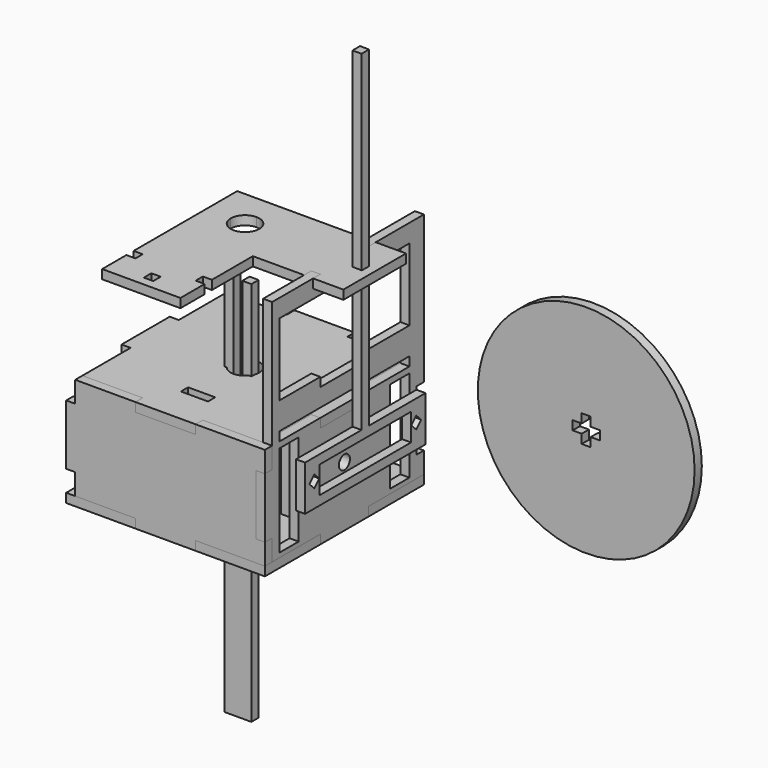
from build123d import *

# Parameters (mm, degrees)
F0_W      = 3
F0_H      = 10
F0_R      = 4.75
F1_DEPTH  = 3
F2_W      = 8
F2_H      = 30.5
F2_R      = 2.3
F2_W_2    = 20
F2_H_2    = 3
F2_W_3    = 3
F2_H_3    = 20
F3_DEPTH  = 3
F5_DEPTH  = 3
F6_R      = 4.75
F6_W      = 20
F6_H      = 3
F6_W_2    = 3
F6_H_2    = 20
F7_DEPTH  = 3
F8_W      = 3
F8_H      = 20
F8_W_2    = 20
F8_H_2    = 3
F8_H_3    = 7
F9_DEPTH  = 3
F10_W     = 17
F10_H     = 20
F10_H_2   = 3
F10_W_2   = 3
F10_W_3   = 3.125
F10_H_3   = 3.125
F10_H_4   = 17
F11_DEPTH = 3
F12_W     = 3.125
F12_H     = 110
F12_W_2   = 6
F12_H_2   = 9
F13_DEPTH = 3
F14_R     = 36
F15_DEPTH = 3
F17_DEPTH = 3
F18_W     = 3
F18_H     = 9
F18_W_2   = 9
F18_H_2   = 3
F19_DEPTH = 37
F20_R     = 2.3
F20_W     = 9
F20_H     = 3
F21_DEPTH = 3


with BuildPart() as f1:
    # F0 (on Top) → F1 (new body)
    with BuildSketch(Plane.XY):
        Polygon((33, 10), (33, 33), (10, 33), (10, 30), (-10, 30), (-10, 33), (-33, 33), (-33, 10), (-30, 10), (-30, -10), (-33, -10), (-33, -33), (-10, -33), (-10, -30), (10, -30), (10, -33), (33, -33), (33, -10), (30, -10), (30, 10), align=None)
        with Locations((-10, 0)):
            Rectangle(F0_W, F0_H, mode=Mode.SUBTRACT)
        Circle(F0_R, mode=Mode.SUBTRACT)
        with Locations((10, 0)):
            Rectangle(F0_W, F0_H, mode=Mode.SUBTRACT)
    extrude(amount=F1_DEPTH)


with BuildPart() as f3:
    # F2 (on face) → F3 (new body)
    with BuildSketch(Plane.YZ.offset(30)):
        Polygon((-30, 10), (-30, 3), (-10, 3), (10, 3), (24, 3), (27, 3), (33, 3), (33, 10), (30, 10), (30, 30), (33, 30), (33, 37), (27, 37), (24, 37), (10, 37), (10, 34), (-10, 34), (-10, 37), (-24, 37), (-27, 37), (-30, 37), (-30, 30), align=None)
        with Locations((-23, 19.75)):
            Rectangle(F2_W, F2_H, mode=Mode.SUBTRACT)
        with Locations((0, 20)):
            Circle(F2_R, mode=Mode.SUBTRACT)
        with Locations((23, 19.75)):
            Rectangle(F2_W, F2_H, mode=Mode.SUBTRACT)
        with Locations((0, 1.5)):
            Rectangle(F2_W_2, F2_H_2)
        with Locations((-31.5, 20)):
            Rectangle(F2_W_3, F2_H_3)
        Polygon((-30, 79), (-30, 49), (-27, 49), (-27, 73), (27, 73), (27, 49), (33, 49), (33, 79), (10, 79), (10, 76), (-10, 76), (-10, 79), align=None)
        Polygon((-30, 49), (-30, 37), (-27, 37), (-27, 40), (27, 40), (27, 37), (33, 37), (33, 49), (27, 49), (10, 49), (10, 46), (-10, 46), (-10, 49), (-27, 49), align=None)
    extrude(amount=F3_DEPTH)


with BuildPart() as f5:
    # F4 (on Front) → F5 (new body)
    with BuildSketch(Plane.XZ):
        Polygon((4.5, -64), (4.5, 64), (1.5, 64), (1.5, 0), (-1.5, 0), (-1.5, 64), (-4.5, 64), (-4.5, -64), align=None)
    extrude(amount=F5_DEPTH)


with BuildPart() as f7:
    # F6 (on face) → F7 (new body)
    with BuildSketch(Plane.XY.offset(34)):
        Polygon((-30, -10), (-30, -30), (-10, -30), (10, -30), (30, -30), (30, -10), (30, 10), (30, 30), (10, 30), (-10, 30), (-30, 30), (-30, 10), align=None)
        Circle(F6_R, mode=Mode.SUBTRACT)
        with Locations((0, -31.5)):
            Rectangle(F6_W, F6_H)
        with Locations((-31.5, 0)):
            Rectangle(F6_W_2, F6_H_2)
        with Locations((31.5, 0)):
            Rectangle(F6_W_2, F6_H_2)
        with Locations((0, 31.5)):
            Rectangle(F6_W, F6_H)
    extrude(amount=F7_DEPTH)


with BuildPart() as f9:
    # F8 (on face) → F9 (new body)
    with BuildSketch(Plane.XZ.offset(30)):
        Polygon((-30, 10), (-30, 3), (-10, 3), (10, 3), (30, 3), (30, 10), (30, 30), (30, 34), (10, 34), (-10, 34), (-10, 37), (-30, 37), (-30, 30), align=None)
        with Locations((-31.5, 20)):
            Rectangle(F8_W, F8_H)
        with Locations((0, 1.5)):
            Rectangle(F8_W_2, F8_H_2)
        with Locations((31.5, 6.5)):
            Rectangle(F8_W, F8_H_3)
        with Locations((20, 35.5)):
            Rectangle(F8_W_2, F8_H_2)
        Polygon((30, 34), (30, 30), (33, 30), (33, 37), (30, 37), align=None)
    extrude(amount=F9_DEPTH)


with BuildPart() as f11:
    # F10 (on face) → F11 (new body)
    with BuildSketch(Plane.XY.offset(76)):
        with Locations((21.5, 0)):
            Rectangle(F10_W, F10_H)
        with Locations((21.5, 11.5)):
            Rectangle(F10_W, F10_H_2)
        with Locations((31.5, 0)):
            Rectangle(F10_W_2, F10_H)
        Polygon((33, 13), (33, 10), (33, -10), (33, -13), (43.0625, -13), (43.0625, 13), align=None)
        with Locations((38.5, 0)):
            Rectangle(F10_W_3, F10_H_3, mode=Mode.SUBTRACT)
        Polygon((13, -10), (13, 10), (10, 10), (10, 0), (10, -10), align=None)
        with Locations((11.5, 11.5)):
            Rectangle(F10_W_2, F10_H_2)
        with Locations((21.5, -11.5)):
            Rectangle(F10_W, F10_H_2)
        with BuildLine():
            Line((10, 0), (10, 10))
            Line((10, 10), (0, 10))
            Line((0, 10), (0, 4.75))
            ThreePointArc((0, 4.75), (3.3587572106, 3.3587572106), (4.75, 0))
            Line((4.75, 0), (10, 0))
        make_face()
        Polygon((0, 10), (10, 10), (10, 13), (-10, 13), (-10, 10), align=None)
        with Locations((11.5, -11.5)):
            Rectangle(F10_W_2, F10_H_2)
        with BuildLine():
            Line((0, 4.75), (0, 10))
            Line((0, 10), (-10, 10))
            Line((-10, 10), (-10, 0))
            Line((-10, 0), (-4.75, 0))
            ThreePointArc((-4.75, 0), (-3.3587572106, 3.3587572106), (0, 4.75))
        make_face()
        with BuildLine():
            Line((10, -10), (10, 0))
            Line((10, 0), (4.75, 0))
            ThreePointArc((4.75, 0), (3.3587572106, -3.3587572106), (0, -4.75))
            Line((0, -4.75), (0, -10))
            Line((0, -10), (10, -10))
        make_face()
        Polygon((10, -13), (10, -10), (0, -10), (-10, -10), (-10, -13), align=None)
        with Locations((11.5, -21.5)):
            Rectangle(F10_W_2, F10_H_4)
        Polygon((-10, 0), (-10, 10), (-13, 10), (-13, -10), (-10, -10), align=None)
        with Locations((-11.5, 11.5)):
            Rectangle(F10_W_2, F10_H_2)
        with BuildLine():
            Line((-10, -10), (0, -10))
            Line((0, -10), (0, -4.75))
            ThreePointArc((0, -4.75), (-3.3587572106, -3.3587572106), (-4.75, 0))
            Line((-4.75, 0), (-10, 0))
            Line((-10, 0), (-10, -10))
        make_face()
        Polygon((10, -30), (10, -13), (-10, -13), (-10, -30), (-10, -33), (10, -33), align=None)
        with Locations((-11.5, -11.5)):
            Rectangle(F10_W_2, F10_H_2)
        with Locations((-11.5, -21.5)):
            Rectangle(F10_W_2, F10_H_4)
        Polygon((13, -33), (10, -33), (-10, -33), (-13, -33), (-13, -43.0625), (13, -43.0625), align=None)
        with Locations((0, -38.5)):
            Rectangle(F10_W_3, F10_H_3, mode=Mode.SUBTRACT)
    extrude(amount=F11_DEPTH)


with BuildPart() as f13:
    # F12 (on face) → F13 (new body)
    with BuildSketch(Plane.YZ.offset(36.9375)):
        with Locations((0, 87.2850484565)):
            Rectangle(F12_W, F12_H)
        Polygon((1.5625, 32.2850484565), (-1.5625, 32.2850484565), (-25, 32.2850484565), (-25, 29.2850484565), (-19, 29.2850484565), (19, 29.2850484565), (25, 29.2850484565), (25, 32.2850484565), align=None)
        with Locations((-22, 24.7850484565)):
            Rectangle(F12_W_2, F12_H_2)
        with Locations((22, 24.7850484565)):
            Rectangle(F12_W_2, F12_H_2)
        Polygon((-19, 20.2850484565), (-25, 20.2850484565), (-25, 17.2850484565), (25, 17.2850484565), (25, 20.2850484565), (19, 20.2850484565), align=None)
    extrude(amount=F13_DEPTH)

    # F16 (on face) → F17 (cut, through all)
    with BuildSketch(Plane.YZ.offset(39.9375)):
        Polygon((-21.1506096654, 23.1838291257), (-19.1, 25.2344387911), (-21.1506096654, 27.2850484565), (-23.2012193309, 25.2344387911), align=None)
        Polygon((21.1506096654, 27.2850484565), (19.1, 25.2344387911), (21.1506096654, 23.1838291257), (23.2012193309, 25.2344387911), align=None)
    extrude(amount=-F17_DEPTH, mode=Mode.SUBTRACT)


with BuildPart() as f15:
    # F14 (on Front) → F15 (new body)
    with BuildSketch(Plane.XZ):
        with Locations((115.7060244211, 57.4378834641)):
            Circle(F14_R)
        Polygon((117.2060244211, 58.9378834641), (120.2060244211, 58.9378834641), (120.2060244211, 55.9378834641), (117.2060244211, 55.9378834641), (117.2060244211, 52.9378834641), (114.2060244211, 52.9378834641), (114.2060244211, 55.9378834641), (111.2060244211, 55.9378834641), (111.2060244211, 58.9378834641), (114.2060244211, 58.9378834641), (114.2060244211, 61.9378834641), (117.2060244211, 61.9378834641), align=None, mode=Mode.SUBTRACT)
    extrude(amount=F15_DEPTH)


with BuildPart() as f19_tool:
    # F18 (on face) → F19 (new body, through all)
    with BuildSketch(Plane.XY.offset(37)):
        with Locations((19.5, 0)):
            Rectangle(F18_W, F18_H)
        with Locations((0, -19.5)):
            Rectangle(F18_W_2, F18_H_2)
    extrude(amount=-F19_DEPTH)


with BuildPart() as f1_1:
    add(f1.part)

    # F19: cut by f19_tool
    add(f19_tool.part, mode=Mode.SUBTRACT)


with BuildPart() as f7_1:
    add(f7.part)

    # F19: cut by f19_tool
    add(f19_tool.part, mode=Mode.SUBTRACT)


with BuildPart() as f21:
    # F20 (on face) → F21 (new body)
    with BuildSketch(Plane(origin=(21, 0, 0), x_dir=(0, -1, 0), z_dir=(-1, 0, 0))):
        Polygon((-7.5, 34), (-7.5, 3), (-4.5, 3), (4.5, 3), (7.5, 3), (7.5, 34), (4.5, 34), (-4.5, 34), align=None)
        with Locations((0, 20)):
            Circle(F20_R, mode=Mode.SUBTRACT)
        with Locations((0, 1.5)):
            Rectangle(F20_W, F20_H)
        with Locations((0, 35.5)):
            Rectangle(F20_W, F20_H)
    extrude(amount=F21_DEPTH)


solid = Compound([f3.part, f5.part, f9.part, f11.part, f13.part, f15.part, f1_1.part, f7_1.part, f21.part])
